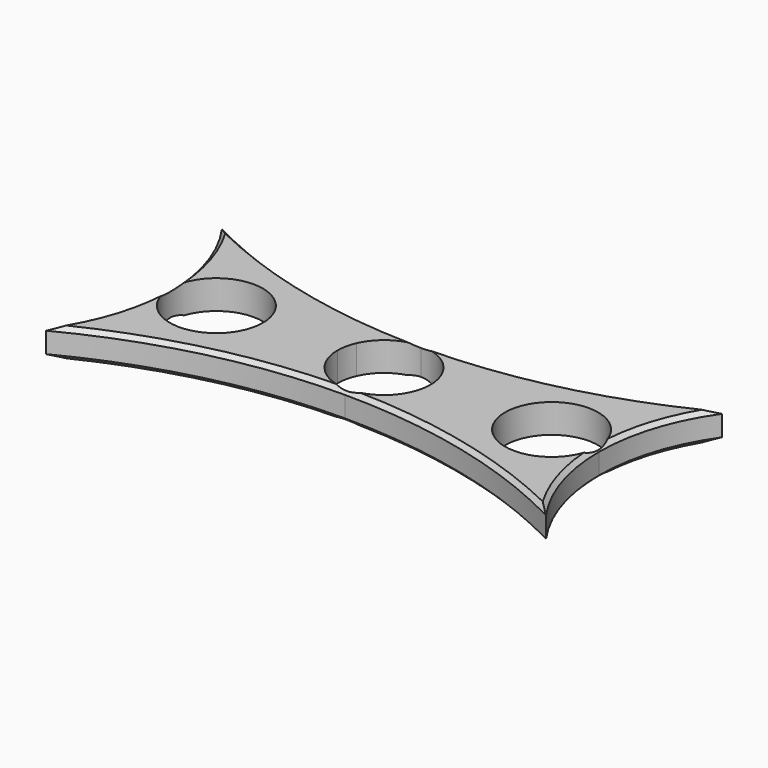
from build123d import *

# Parameters (mm, degrees)
F1_DEPTH     = 7
F2_T2_ANGLE  = 57.1143931605
F2_T4_ANGLE  = 57.1143931605
F2_T6_ANGLE  = 76.6293726343
F2_T8_ANGLE  = 76.6293726343
F2_T10_ANGLE = 57.1143931605
F2_T12_ANGLE = 76.6293726343
F2_T14_ANGLE = 76.6293726343
F2_T16_ANGLE = 57.1143931605


# Not quite as in the source:
# - a fillet or chamfer that OpenCascade refuses, or shapes differently, is made with other operations: its cross-section is extruded or revolved along the edge and cut away or added


with BuildPart() as f1:
    # F0 (on Top) → F1 (new body)
    with BuildSketch(Plane.XY):
        with BuildLine():
            ThreePointArc((-51.9588312409, 22.6017753357), (-59.8237606638, 25.7612832302), (-67.4684691244, 29.4216162089))
            ThreePointArc((-67.4684691244, 29.4216162089), (-61.2035945552, 16.7707381256), (-59.0483218899, 2.8191013262))
            Line((-59.0483218899, 2.8191013262), (-58.7843277942, 2.8191013262))
            ThreePointArc((-58.7843277942, 2.8191013262), (-47.5343277942, 14.0691013262), (-36.2843277942, 2.8191013262))
            Line((-36.2843277942, 2.8191013262), (-18.2192023098, 2.8191013262))
            ThreePointArc((-18.2192023098, 2.8191013262), (-17.978724805, 5.1327379505), (-17.267573078, 7.3474630081))
            Line((-17.267573078, 7.3474630081), (-51.9588312409, 22.6017753357))
        make_face()
        with BuildLine():
            ThreePointArc((-6.9692023098, 14.6539675384), (-29.8123323501, 16.6561845448), (-51.9588312409, 22.6017753357))
            Line((-51.9588312409, 22.6017753357), (-17.267573078, 7.3474630081))
            ThreePointArc((-17.267573078, 7.3474630081), (-13.1181221775, 12.2399974863), (-6.9692023098, 14.0691013262))
            Line((-6.9692023098, 14.0691013262), (-6.9692023098, 14.6539675384))
        make_face()
        with BuildLine():
            Line((-58.7843277942, 2.8191013262), (-59.0483218899, 2.8191013262))
            ThreePointArc((-59.0483218899, 2.8191013262), (-61.2035945552, -11.1325354733), (-67.4684691244, -23.7834135565))
            ThreePointArc((-67.4684691244, -23.7834135565), (-38.1069797367, -12.7610910953), (-6.9692023098, -9.0157648861))
            Line((-6.9692023098, -9.0157648861), (-6.9692023098, -8.4308986738))
            ThreePointArc((-6.9692023098, -8.4308986738), (-14.9241535982, -5.1358499622), (-18.2192023098, 2.8191013262))
            Line((-18.2192023098, 2.8191013262), (-36.2843277942, 2.8191013262))
            ThreePointArc((-36.2843277942, 2.8191013262), (-47.5343277942, -8.4308986738), (-58.7843277942, 2.8191013262))
        make_face()
        with BuildLine():
            ThreePointArc((45.1099172702, 2.8191013262), (47.2651899355, 16.7707381256), (53.5300645047, 29.4216162089))
            ThreePointArc((53.5300645047, 29.4216162089), (24.168575117, 18.3992937476), (-6.9692023098, 14.6539675384))
            Line((-6.9692023098, 14.6539675384), (-6.9692023098, 14.0691013262))
            ThreePointArc((-6.9692023098, 14.0691013262), (0.9857489785, 10.7740526145), (4.2807976902, 2.8191013262))
            Line((4.2807976902, 2.8191013262), (22.3459231745, 2.8191013262))
            ThreePointArc((22.3459231745, 2.8191013262), (33.5959231745, 14.0691013262), (44.8459231745, 2.8191013262))
            Line((44.8459231745, 2.8191013262), (45.1099172702, 2.8191013262))
        make_face()
        with BuildLine():
            ThreePointArc((53.5300645047, -23.7834135565), (47.2651899355, -11.1325354733), (45.1099172702, 2.8191013262))
            Line((45.1099172702, 2.8191013262), (44.8459231745, 2.8191013262))
            ThreePointArc((44.8459231745, 2.8191013262), (33.5959231745, -8.4308986738), (22.3459231745, 2.8191013262))
            Line((22.3459231745, 2.8191013262), (4.2807976902, 2.8191013262))
            ThreePointArc((4.2807976902, 2.8191013262), (4.0403201853, 0.5054647019), (3.3291684583, -1.7092603557))
            Line((3.3291684583, -1.7092603557), (38.0204266212, -16.9635726834))
            ThreePointArc((38.0204266212, -16.9635726834), (45.8853560441, -20.1230805779), (53.5300645047, -23.7834135565))
        make_face()
        with BuildLine():
            Line((-6.9692023098, -8.4308986738), (-6.9692023098, -9.0157648861))
            ThreePointArc((-6.9692023098, -9.0157648861), (15.8739277304, -11.0179818925), (38.0204266212, -16.9635726834))
            Line((38.0204266212, -16.9635726834), (3.3291684583, -1.7092603557))
            ThreePointArc((3.3291684583, -1.7092603557), (-0.8202824422, -6.601794834), (-6.9692023098, -8.4308986738))
        make_face()
    extrude(amount=F1_DEPTH)

    # F2: chamfer of 1 on 8 edges, made by hand

    # F2_s1 → F2_t2 (revolve, cut)
    with BuildSketch(Plane(origin=(-64.2958342843, -34.9929409524, 0), x_dir=(0, 0, 1), z_dir=(-0.8783403422, -0.4780358179, 0))):
        Polygon((6, 11.3876031391), (7, 12.3876031391), (7, 11.3876031391), align=None)
    revolve(axis=Axis((-6.9692023098, -140.3245743959, 7), (0, 0, -1)), revolution_arc=F2_T2_ANGLE, mode=Mode.SUBTRACT)

    # F2_s3 → F2_t4 (revolve, cut)
    with BuildSketch(Plane(origin=(55.9099674663, 30.4289416566, 0), x_dir=(0, 0, 1), z_dir=(0.8783403422, 0.4780358179, 0))):
        Polygon((6, -0.2277143611), (7, 0.7722856389), (7, -0.2277143611), align=None)
    revolve(axis=Axis((-6.9692023098, 145.9627770483, 7), (0, 0, -1)), revolution_arc=F2_T4_ANGLE, mode=Mode.SUBTRACT)

    # F2_s5 → F2_t6 (revolve, cut)
    with BuildSketch(Plane(origin=(-41.8392456248, 52.9497637497, 0), x_dir=(0, 0, 1), z_dir=(-0.6199801689, 0.7846174801, 0))):
        Polygon((6, -34.6245823345), (7, -33.6245823345), (7, -34.6245823345), align=None)
    revolve(axis=Axis((-105.2822329994, 2.8191013262, 7), (0, 0, -1)), revolution_arc=F2_T6_ANGLE, mode=Mode.SUBTRACT)

    # F2_s7 → F2_t8 (revolve, cut)
    with BuildSketch(Plane(origin=(-41.8392456248, 52.9497637497, 0), x_dir=(0, 0, 1), z_dir=(-0.6199801689, 0.7846174801, 0))):
        Polygon((1, -34.6245823345), (0, -33.6245823345), (0, -34.6245823345), align=None)
    revolve(axis=Axis((-105.2822329994, 2.8191013262, 0), (0, 0, -1)), revolution_arc=F2_T8_ANGLE, mode=Mode.SUBTRACT)

    # F2_s9 → F2_t10 (revolve, cut)
    with BuildSketch(Plane(origin=(55.9099674663, 30.4289416566, 0), x_dir=(0, 0, 1), z_dir=(0.8783403422, 0.4780358179, 0))):
        Polygon((1, -0.2277143611), (0, 0.7722856389), (0, -0.2277143611), align=None)
    revolve(axis=Axis((-6.9692023098, 145.9627770483, 0), (0, 0, -1)), revolution_arc=F2_T10_ANGLE, mode=Mode.SUBTRACT)

    # F2_s11 → F2_t12 (revolve, cut)
    with BuildSketch(Plane(origin=(33.7389773041, -42.6984485674, 0), x_dir=(0, 0, 1), z_dir=(0.6199801689, -0.7846174801, 0))):
        Polygon((1, -27.1838402573), (0, -26.1838402573), (0, -27.1838402573), align=None)
    revolve(axis=Axis((91.3438283797, 2.8191013262, 0), (0, 0, -1)), revolution_arc=F2_T12_ANGLE, mode=Mode.SUBTRACT)

    # F2_s13 → F2_t14 (revolve, cut)
    with BuildSketch(Plane(origin=(33.7389773041, -42.6984485674, 0), x_dir=(0, 0, 1), z_dir=(0.6199801689, -0.7846174801, 0))):
        Polygon((6, -27.1838402573), (7, -26.1838402573), (7, -27.1838402573), align=None)
    revolve(axis=Axis((91.3438283797, 2.8191013262, 7), (0, 0, -1)), revolution_arc=F2_T14_ANGLE, mode=Mode.SUBTRACT)

    # F2_s15 → F2_t16 (revolve, cut)
    with BuildSketch(Plane(origin=(-64.2958342843, -34.9929409524, 0), x_dir=(0, 0, 1), z_dir=(-0.8783403422, -0.4780358179, 0))):
        Polygon((1, 11.3876031391), (0, 12.3876031391), (0, 11.3876031391), align=None)
    revolve(axis=Axis((-6.9692023098, -140.3245743959, 0), (0, 0, -1)), revolution_arc=F2_T16_ANGLE, mode=Mode.SUBTRACT)


solid = f1.part
